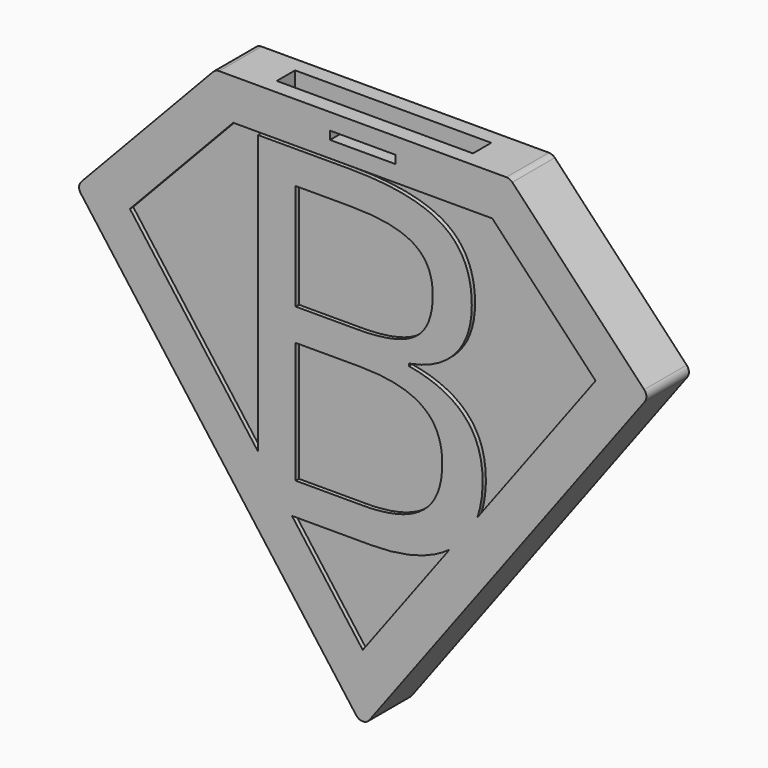
from build123d import *

# Parameters (mm, degrees)
F1_DEPTH     = 3.25
F3_DEPTH     = 0.5
F5_DEPTH     = 0.5
F6_TEXT_SIZE = 55.5555555556
F7_DEPTH     = 0.5
F8_TEXT_SIZE = 55.5555555556
F9_DEPTH     = 0.5
F10_W        = 24
F10_H        = 2.8
F11_DEPTH    = 20
F13_DEPTH    = 1.4
F14_W        = 8
F14_H        = 1
F15_DEPTH    = 25
F16_R        = 1


# Not quite as in the source:
# - Text() gives the source's letters only with a copy of the font that has no kerning and outlines rounded to 1/6400 em; it was checked with that copy


with BuildPart() as f1:
    # F0 (on Front) → F1 (new body, symmetric)
    with BuildSketch(Plane.XZ):
        Polygon((18, 18), (0, 18), (-18, 18), (-35, 0), (0, -47), (35, 0), align=None)
    extrude(amount=F1_DEPTH, both=True)

    # F2 (on face) → F3 (cut)
    with BuildSketch(Plane.XZ.offset(3.25)):
        Polygon((15.8447675538, 13), (-15.8447675538, 13), (-28.4822773709, -0.3808927475), (1.162e-07, -38.628522516), (28.4822775009, -0.3808928851), align=None)
    extrude(amount=-F3_DEPTH, mode=Mode.SUBTRACT)

    # F4 (on face) → F5 (cut)
    with BuildSketch(Plane(origin=(0, 3.25, 0), x_dir=(-1, 0, 0), z_dir=(0, 1, 0))):
        Polygon((28.482277527, -0.3808925379), (15.8447676545, 13.0000002682), (-15.8447670441, 13.0000002682), (-28.4822772579, -0.3808928993), (0, -38.6285223599), align=None)
    extrude(amount=-F5_DEPTH, mode=Mode.SUBTRACT)

    # F6 (on face) → F7 (join)
    with BuildSketch(Plane.XZ.offset(2.75)):
        with Locations((-18.2682291667, -27)):
            Text('B', F6_TEXT_SIZE, font='Open Sans', text_align=(TextAlign.LEFT, TextAlign.BOTTOM))
    extrude(amount=F7_DEPTH)

    # F8 (on face) → F9 (join)
    with BuildSketch(Plane(origin=(0, 2.75, 0), x_dir=(-1, 0, 0), z_dir=(0, 1, 0))):
        with Locations((-18.2682291667, -26.9999997318)):
            Text('B', F8_TEXT_SIZE, font='Open Sans', text_align=(TextAlign.LEFT, TextAlign.BOTTOM))
    extrude(amount=F9_DEPTH)

    # F10 (on face) → F11 (cut)
    with BuildSketch(Plane.XY.offset(18)):
        Rectangle(F10_W, F10_H)
    extrude(amount=-F11_DEPTH, mode=Mode.SUBTRACT)

    # F12 (on Front) → F13 (cut, symmetric)
    with BuildSketch(Plane.XZ):
        with BuildLine():
            Line((12, -2), (-12, -2))
            ThreePointArc((-12, -2), (0, -14), (12, -2))
        make_face()
    extrude(amount=F13_DEPTH, both=True, mode=Mode.SUBTRACT)

    # F14 (on face) → F15 (cut)
    with BuildSketch(Plane.XZ.offset(3.25)):
        with Locations((0, 15.5)):
            Rectangle(F14_W, F14_H)
    extrude(amount=-F15_DEPTH, mode=Mode.SUBTRACT)

    # F16
    f16_edges = [f1.edges().sort_by_distance(p)[0] for p in [
        (0, 0, -47),
        (35, 0, 0),
        (-35, 0, 0),
        (-18, 0, 18),
        (18, 0, 18),
    ]]
    fillet(f16_edges, radius=F16_R)


solid = f1.part
